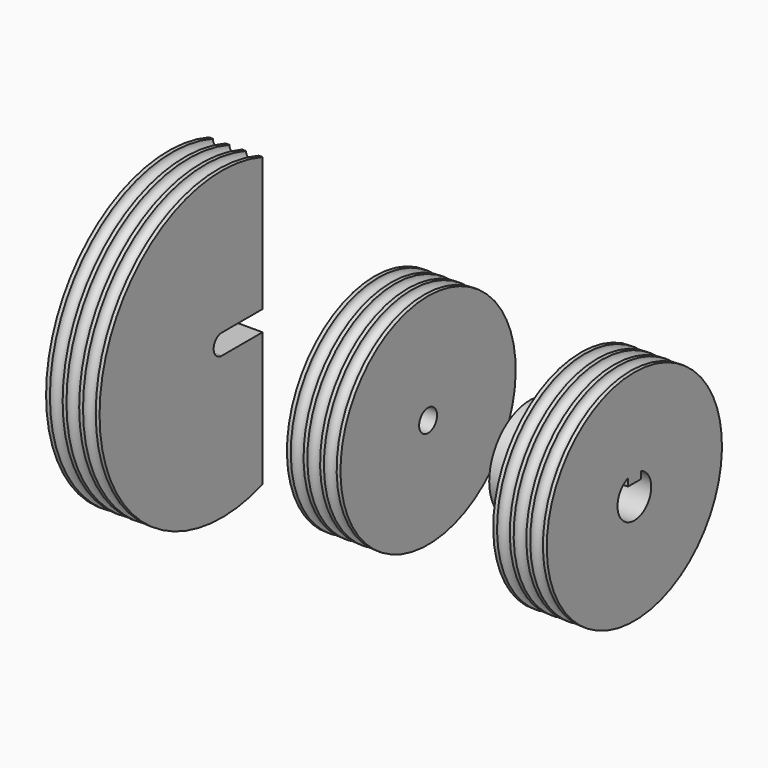
from build123d import *

# Parameters (mm, degrees)
F2_R      = 2.794
F3_DEPTH  = 64.7707550396
F5_DEPTH  = 25.4
F6_R      = 12.7
F7_DEPTH  = 12.7
F9_DEPTH  = 13.3358775198
F10_DEPTH = 25.4


# Not quite as in the source:
# - ends of sketch curves that miss each other by under 0.0002 mm in the source are joined
# - a feature names something its author has since deleted; it is built from what else it names


with BuildPart() as f1:
    # F0 (on Front) → F1 (revolve)
    with BuildSketch(Plane.XZ):
        with BuildLine():
            ThreePointArc((-9.2074912607, 27.305), (-10.8044939562, 25.7175284416), (-12.3823774954, 27.3240050505))
            Line((-12.3823774954, 27.3240050505), (-13.3348775198, 27.3240050505))
            Line((-13.3348775198, 27.3240050505), (-13.3348775198, 0))
            Line((-13.3348775198, 0), (0, 0))
            Line((0, 0), (0, 27.305))
            Line((0, 27.305), (-0.9524999854, 27.305))
            ThreePointArc((-0.9524999854, 27.305), (-2.5399912119, 25.7175), (-4.1274912119, 27.305))
            Line((-4.1274912119, 27.305), (-5.0799912363, 27.305))
            ThreePointArc((-5.0799912363, 27.305), (-6.6674912363, 25.7175), (-8.2549912363, 27.305))
            Line((-8.2549912363, 27.305), (-9.2074912607, 27.305))
        make_face()
    revolve(axis=Axis((-6.6674387599, 0, 0), (1, 0, 0)))

    # F2 (on face) → F3 (cut, through all)
    with BuildSketch(Plane.YZ):
        Circle(F2_R)
    extrude(amount=-F3_DEPTH, mode=Mode.SUBTRACT)


with BuildPart() as f1b:
    # F0 (on Front) → F1, piece 2 (revolve)
    with BuildSketch(Plane.XZ):
        with BuildLine():
            ThreePointArc((42.2273862591, 27.305), (40.6306157957, 25.7175270684), (39.0524945318, 27.3235406107))
            Line((39.0524945318, 27.3235406107), (38.1, 27.3235406107))
            Line((38.1, 27.3235406107), (38.1, 0))
            Line((38.1, 0), (51.4348776012, 0))
            Line((51.4348776012, 0), (51.4348776012, 27.305))
            Line((51.4348776012, 27.305), (50.4823743203, 27.305))
            ThreePointArc((50.4823743203, 27.305), (48.8948753228, 25.7175), (47.3073753228, 27.305))
            Line((47.3073753228, 27.305), (46.3548807909, 27.305))
            ThreePointArc((46.3548807909, 27.305), (44.7673807909, 25.7175), (43.1798807909, 27.305))
            Line((43.1798807909, 27.305), (42.2273862591, 27.305))
        make_face()
    revolve(axis=Axis((-6.6674387599, 0, 0), (1, 0, 0)))

    # F4 (on face) → F5 (cut)
    with BuildSketch(Plane.YZ.offset(51.4348776012)):
        with BuildLine():
            Line((-2, 3), (-2, 4.8584479003))
            ThreePointArc((-2, 4.8584479003), (0, -5.254), (2, 4.8584479003))
            Line((2, 4.8584479003), (2, 3))
            Line((2, 3), (-2, 3))
        make_face()
    extrude(amount=-F5_DEPTH, mode=Mode.SUBTRACT)

    # F6 (on face) → F7 (join)
    with BuildSketch(Plane(origin=(38.1, 0, 0), x_dir=(0, -1, 0), z_dir=(-1, 0, 0))):
        Circle(F6_R)
        with BuildLine():
            ThreePointArc((2, 4.8584479003), (0, -5.254), (-2, 4.8584479003))
            Line((-2, 4.8584479003), (-2, 3))
            Line((-2, 3), (2, 3))
            Line((2, 3), (2, 4.8584479003))
        make_face(mode=Mode.SUBTRACT)
    extrude(amount=F7_DEPTH)


with BuildPart() as f1c:
    # F0 (on Front) → F1, piece 3 (revolve)
    with BuildSketch(Plane.XZ):
        with BuildLine():
            ThreePointArc((-56.5147550884, 38.099999532), (-58.102255298, 36.5125000244), (-59.6897550396, 38.1))
            Line((-59.6897550396, 38.1), (-60.642255064, 38.1))
            ThreePointArc((-60.642255064, 38.1), (-62.2297550396, 36.5125000244), (-63.8172550152, 38.1))
            Line((-63.8172550152, 38.1), (-64.7697550396, 38.1))
            Line((-64.7697550396, 38.1), (-64.7697550396, 0))
            Line((-64.7697550396, 0), (-51.4348775198, 0))
            Line((-51.4348775198, 0), (-51.4348775198, 38.1))
            Line((-51.4348775198, 38.1), (-52.3873775442, 38.1))
            ThreePointArc((-52.3873775442, 38.1), (-53.9748775198, 36.5125000244), (-55.5623774954, 38.1))
            Line((-55.5623774954, 38.1), (-56.5147550884, 38.099999532))
        make_face()
    revolve(axis=Axis((-6.6674387599, 0, 0), (1, 0, 0)))

    # F8 (on face) → F9 (cut, through all)
    with BuildSketch(Plane.YZ.offset(-51.4348775198)):
        with BuildLine():
            Line((12.7, 35.9210244843), (12.7, 2.54))
            Line((12.7, 2.54), (12.7, -2.54))
            Line((12.7, -2.54), (12.7, -35.9210244843))
            ThreePointArc((12.7, -35.9210244843), (31.1085197333, -21.9970452561), (38.1, 0))
            ThreePointArc((38.1, 0), (31.1085197333, 21.9970452561), (12.7, 35.9210244843))
        make_face()
    extrude(amount=-F9_DEPTH, mode=Mode.SUBTRACT)

    # F8 (on face) → F10 (cut)
    with BuildSketch(Plane.YZ.offset(-51.4348775198)):
        with BuildLine():
            ThreePointArc((0, -2.54), (1.7960512242, -1.7960512242), (2.54, 0))
            ThreePointArc((2.54, 0), (1.7960512242, 1.7960512242), (0, 2.54))
            ThreePointArc((0, 2.54), (-2.54, 0), (0, -2.54))
        make_face()
        with BuildLine():
            ThreePointArc((0, 2.54), (1.7960512242, 1.7960512242), (2.54, 0))
            ThreePointArc((2.54, 0), (1.7960512242, -1.7960512242), (0, -2.54))
            Line((0, -2.54), (12.7, -2.54))
            Line((12.7, -2.54), (12.7, 2.54))
            Line((12.7, 2.54), (0, 2.54))
        make_face()
    extrude(amount=-F10_DEPTH, mode=Mode.SUBTRACT)


solid = Compound([f1.part, f1b.part, f1c.part])
